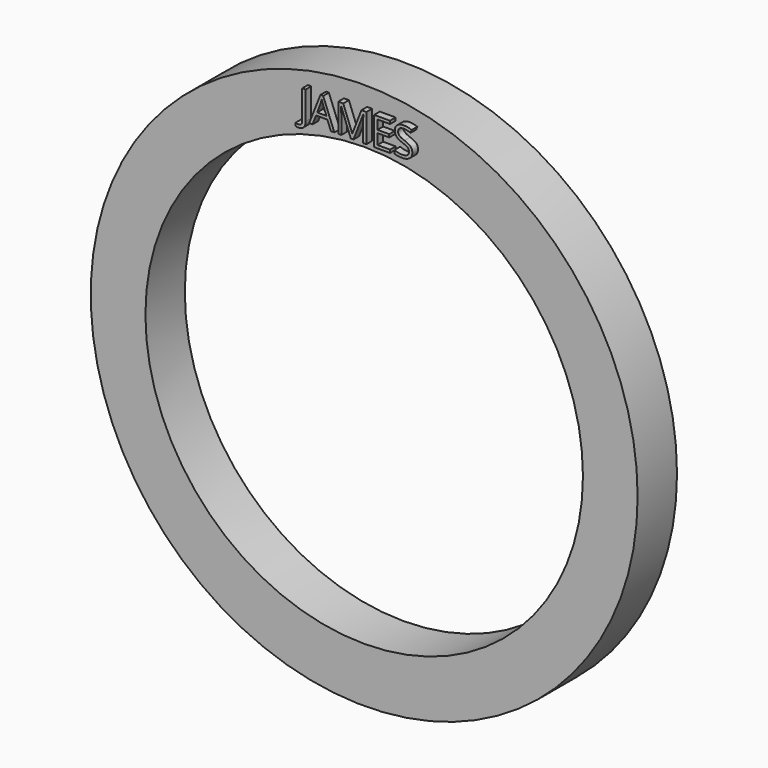
from build123d import *

# Parameters (mm, degrees)
F0_R         = 50
F0_R_2       = 40
F1_DEPTH     = 9
F2_TEXT_SIZE = 7.273712092
F3_DEPTH     = 1.3


# Not quite as in the source:
# - Text() gives the source's letters only with a copy of the font that has no kerning and outlines rounded to 1/6400 em; it was checked with that copy


with BuildPart() as f1:
    # F0 (on Front) → F1 (new body)
    with BuildSketch(Plane.XZ):
        Circle(F0_R)
        Circle(F0_R_2, mode=Mode.SUBTRACT)
    extrude(amount=F1_DEPTH)

    # F2 (on face) → F3 (join)
    with BuildSketch(Plane.XZ.offset(9)):
        with Locations((-10.9590525972, 41.4116457105)):
            Text('JAMES', F2_TEXT_SIZE, font='Open Sans', text_align=(TextAlign.LEFT, TextAlign.BOTTOM))
    extrude(amount=F3_DEPTH)


solid = f1.part
